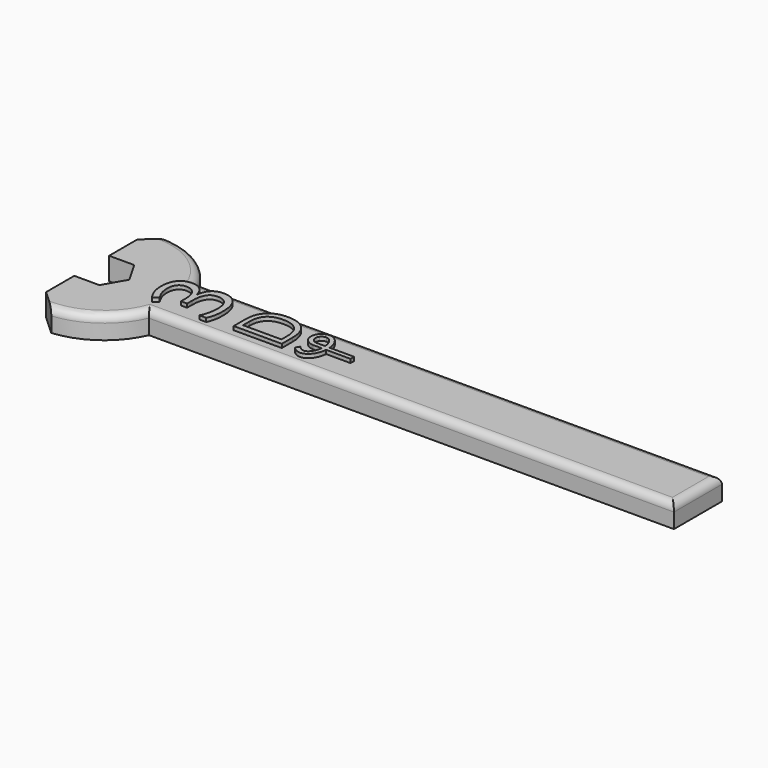
from build123d import *

# Parameters (mm, degrees)
F1_DEPTH       = 3
F2_T1_DEPTH    = 16.236004638
F3_R           = 1
F4_TEXT_SIZE   = 11.6930572473
F4_TEXT_SIZE_2 = 8.9824561404
F5_DEPTH       = 0.5
F7_DEPTH       = 0.5


# Not quite as in the source:
# - a fillet or chamfer that OpenCascade refuses, or shapes differently, is made with other operations: its cross-section is extruded or revolved along the edge and cut away or added
# - Text() gives the source's letters only with a copy of the font that has no kerning and outlines rounded to 1/6400 em; it was checked with that copy


with BuildPart() as f1:
    # F0 (on Top) → F1 (new body)
    with BuildSketch(Plane.XY):
        with BuildLine():
            Line((-1.6743157806, 9.8588369835), (-1.6743157806, 2.9))
            Line((-1.6743157806, 2.9), (1.6743157806, 2.9))
            Line((1.6743157806, 2.9), (3.3486315613, 0))
            Line((3.3486315613, 0), (1.6743157806, -2.9))
            Line((1.6743157806, -2.9), (-1.6743157806, -2.9))
            Line((-1.6743157806, -2.9), (-1.6743157806, -9.8588369835))
            ThreePointArc((-1.6743157806, -9.8588369835), (4.7549602765, -8.7971786823), (9.1651513899, -4))
            Line((9.1651513899, -4), (79.1651513899, -4))
            Line((79.1651513899, -4), (79.1651513899, 4))
            Line((79.1651513899, 4), (9.1651513899, 4))
            ThreePointArc((9.1651513899, 4), (4.7549602765, 8.7971786823), (-1.6743157806, 9.8588369835))
        make_face()
    extrude(amount=F1_DEPTH)

    # F2: chamfer of 2 on 2 edges, made by hand

    # F2_s2 → F2_t1 (cut)
    with BuildSketch(Plane.XY.offset(-6.618002319)):
        with BuildLine():
            Line((0.96842124, -10.0125047778), (-1.7334003618, -7.5461514983))
            Line((-1.7334003618, -7.5461514983), (-1.7734003618, -7.5461514983))
            ThreePointArc((-1.7734003618, -7.5461514983), (-1.7143157806, -8.7024942409), (-1.7143157806, -9.8588369835))
            Line((-1.7143157806, -9.8588369835), (-1.6810130438, -9.8982723314))
            ThreePointArc((-1.6810130438, -9.8982723314), (-0.3564285613, -10.0336712464), (0.9720585866, -10.0523390559))
            Line((0.9720585866, -10.0523390559), (0.96842124, -10.0125047778))
        make_face()
        with BuildLine():
            Line((0.96842124, 10.0125047778), (-1.7334003618, 7.5461514983))
            Line((-1.7334003618, 7.5461514983), (-1.7734003618, 7.5461514983))
            ThreePointArc((-1.7734003618, 7.5461514983), (-1.7143157806, 8.7024942409), (-1.7143157806, 9.8588369835))
            Line((-1.7143157806, 9.8588369835), (-1.6810130438, 9.8982723314))
            ThreePointArc((-1.6810130438, 9.8982723314), (-0.3564285613, 10.0336712464), (0.9720585866, 10.0523390559))
            Line((0.9720585866, 10.0523390559), (0.96842124, 10.0125047778))
        make_face()
    extrude(amount=F2_T1_DEPTH, mode=Mode.SUBTRACT)

    # F3
    f3_edges = [f1.edges().sort_by_distance(p)[0] for p in [
        (5.852347, 8.10864, 3),
        (44.165151, -4, 3),
        (44.165151, 4, 3),
        (79.165151, 0, 3),
        (5.852347, -8.10864, 3),
    ]]
    fillet(f3_edges, radius=F3_R)

    # F4 (on face) → F5 (join)
    with BuildSketch(Plane.XY.offset(3)):
        with Locations(Location((15.9042825923, -3), (0, 0, 90))):
            Text('3', F4_TEXT_SIZE, font='Open Sans', text_align=(TextAlign.LEFT, TextAlign.BOTTOM))
        with Locations(Location((25.3716510133, -3), (0, 0, 90))):
            Text('D', F4_TEXT_SIZE_2, font='Open Sans', text_align=(TextAlign.LEFT, TextAlign.BOTTOM))
    extrude(amount=F5_DEPTH)

    # F6 (on face) → F7 (join)
    with BuildSketch(Plane.XY.offset(3)):
        with BuildLine():
            Line((33.0898860097, 0.3), (29.8272403201, 0.3))
            add(Edge.make_bspline(
                [(29.8272403201, -0.3), (29.8526237435, 0), (29.8272403201, 0.3)],
                knots=[4.592099098, 4.592099098, 4.592099098, 4.8326788628, 4.8326788628, 4.8326788628], degree=2, weights=[1, 0.9927738917, 1]))
            Line((29.8272403201, -0.3), (33.0898860097, -0.3))
            Line((33.0898860097, -0.3), (33.0898860097, 0.3))
        make_face()
        with BuildLine():
            Line((29.8272403201, 0.3), (29.2254603515, 0.3))
            add(Edge.make_bspline(
                [(29.2254603515, -0.3), (29.2544949228, 0), (29.2254603515, 0.3)],
                knots=[4.5538306997, 4.5538306997, 4.5538306997, 4.870947261, 4.870947261, 4.870947261], degree=2, weights=[1, 0.9874559494, 1]))
            Line((29.2254603515, -0.3), (29.8272403201, -0.3))
            add(Edge.make_bspline(
                [(29.8272403201, -0.3), (29.8526237435, 0), (29.8272403201, 0.3)],
                knots=[4.592099098, 4.592099098, 4.592099098, 4.8326788628, 4.8326788628, 4.8326788628], degree=2, weights=[1, 0.9927738917, 1]))
        make_face()
        with BuildLine():
            Line((29.2254603515, 0.3), (28.0898860097, 0.3))
            Line((28.0898860097, 0.3), (28.0898860097, 0))
            Line((28.0898860097, 0), (28.0898860097, -0.3))
            Line((28.0898860097, -0.3), (29.2254603515, -0.3))
            add(Edge.make_bspline(
                [(29.2254603515, -0.3), (29.2544949228, 0), (29.2254603515, 0.3)],
                knots=[4.5538306997, 4.5538306997, 4.5538306997, 4.870947261, 4.870947261, 4.870947261], degree=2, weights=[1, 0.9874559494, 1]))
        make_face()
        with BuildLine():
            Line((28.0898860097, -0.3), (28.0898860097, 0))
            Line((28.0898860097, 0), (27.9224803223, -0.289955156))
            ThreePointArc((27.9224803223, -0.289955156), (28.0060326212, -0.2974865328), (28.0898860097, -0.3))
        make_face()
        with BuildLine():
            add(Edge.make_bspline(
                [(29.2254603515, 0.3), (29.0706093049, 1.9), (28.0898860097, 1.9)],
                knots=[4.870947261, 4.870947261, 4.870947261, 6.2831853072, 6.2831853072, 6.2831853072], degree=2, weights=[1, 0.7608859103, 1]))
            Line((29.2254603515, 0.3), (29.8272403201, 0.3))
            add(Edge.make_bspline(
                [(29.8272403201, 0.3), (29.6410952154, 2.5), (28.0898860097, 2.5)],
                knots=[4.8326788628, 4.8326788628, 4.8326788628, 6.2831853072, 6.2831853072, 6.2831853072], degree=2, weights=[1, 0.7483314774, 1]))
            add(Edge.make_bspline(
                [(28.0898860097, 2.5), (27.3918774789, 2.5), (26.885479133, 1.8137254902)],
                knots=[0, 0, 0, 0.759049946, 0.759049946, 0.759049946], degree=2, weights=[1, 0.928840728, 1]))
            ThreePointArc((26.885479133, 1.8137254902), (26.6912364661, 1.0385227342), (26.9527462695, 0.283352456))
            add(Edge.make_bspline(
                [(27.4438995332, 1.5719125683), (27.0277595326, 1.1050962549), (26.9527462695, 0.283352456)],
                knots=[0.5964722291, 0.5964722291, 0.5964722291, 1.4211050472, 1.4211050472, 1.4211050472], degree=2, weights=[1, 0.9161950209, 1]))
            ThreePointArc((27.4438995332, 1.5719125683), (27.7276223313, 1.813277665), (28.0898860097, 1.9))
        make_face()
        with BuildLine():
            Line((28.0898860097, 0), (28.0898860097, 0.3))
            ThreePointArc((28.0898860097, 0.3), (27.3766083447, 0.7377363216), (27.4438995332, 1.5719125683))
            add(Edge.make_bspline(
                [(27.4438995332, 1.5719125683), (27.0277595326, 1.1050962549), (26.9527462695, 0.283352456)],
                knots=[0.5964722291, 0.5964722291, 0.5964722291, 1.4211050472, 1.4211050472, 1.4211050472], degree=2, weights=[1, 0.9161950209, 1]))
            ThreePointArc((26.9527462695, 0.283352456), (27.3774043624, -0.1051431045), (27.9224803223, -0.289955156))
            Line((27.9224803223, -0.289955156), (28.0898860097, 0))
        make_face()
        with BuildLine():
            Line((29.8272403201, -0.3), (29.2254603515, -0.3))
            add(Edge.make_bspline(
                [(27.2961273638, -1.3748303036), (28.8798731628, -3.8707831116), (29.2254603515, -0.3)],
                knots=[2.3797928246, 2.3797928246, 2.3797928246, 4.5538306997, 4.5538306997, 4.5538306997], degree=2, weights=[1, 0.4651263981, 1]))
            Line((27.2961273638, -1.3748303036), (26.9763876745, -1.9286356907))
            add(Edge.make_bspline(
                [(26.9763876745, -1.9286356907), (29.4434827606, -4.835529593), (29.8272403201, -0.3)],
                knots=[2.451919897, 2.451919897, 2.451919897, 4.592099098, 4.592099098, 4.592099098], degree=2, weights=[1, 0.4800456295, 1]))
        make_face()
    extrude(amount=F7_DEPTH)


solid = f1.part
